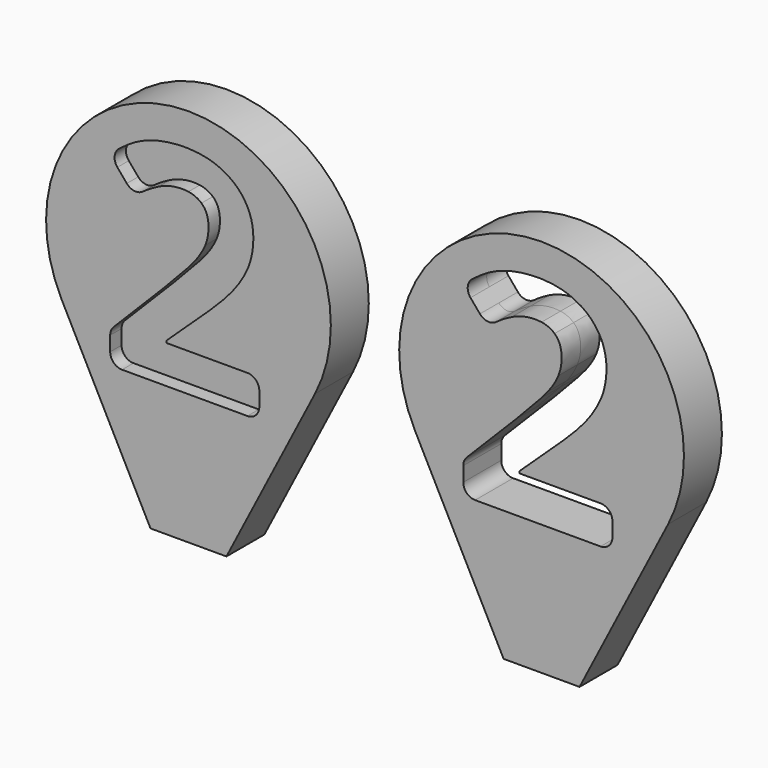
from build123d import *

# Parameters (mm, degrees)
F1_DEPTH = 3.175
F2_R     = 1.5875
F0_W     = 9.4800787622
F0_H     = 5.0789482924
F4_DEPTH = 1.27


with BuildPart() as f1:
    # F0 (on Front) → F1 (new body, symmetric)
    with BuildSketch(Plane.XZ):
        with BuildLine():
            ThreePointArc((-16.9370236714, 23.0299237874), (-9.919300584, 15.486237338), (0, 12.7))
            Line((0, 12.7), (0, 17.4584717806))
            Line((0, 17.4584717806), (-10.4733786127, 17.4584717806))
            Line((-10.4733786127, 17.4584717806), (-10.4733786127, 21.6565692621))
            Line((-10.4733786127, 21.6565692621), (-3.3078759174, 28.897037984))
            add(Edge.make_bspline(
                [(-3.3078759174, 28.897037984), (-1.1437844149, 31.1120492865), (0, 32.4033079857)],
                knots=[0, 0, 0, 0.6792383492, 0.6792383492, 0.6792383492], degree=2))
            Line((0, 32.4033079857), (0, 41.314116363))
            add(Edge.make_bspline(
                [(0, 41.314116363), (-0.3731620425, 41.3726342199), (-0.7902668622, 41.3726342199)],
                knots=[0.7360987537, 0.7360987537, 0.7360987537, 1, 1, 1], degree=2))
            add(Edge.make_bspline(
                [(-0.7902668622, 41.3726342199), (-2.4457666131, 41.3726342199), (-4.0075588309, 40.6104796177)],
                knots=[0, 0, 0, 1, 1, 1], degree=2))
            add(Edge.make_bspline(
                [(-4.0075588309, 40.6104796177), (-5.5693510488, 39.8483250154), (-7.2685809818, 38.4427120193)],
                knots=[0, 0, 0, 1, 1, 1], degree=2))
            Line((-7.2685809818, 38.4427120193), (-10.5483446392, 42.3284510573))
            add(Edge.make_bspline(
                [(-10.5483446392, 42.3284510573), (-8.4430487296, 44.1276356922), (-7.0561772401, 44.8679252034)],
                knots=[0, 0, 0, 1, 1, 1], degree=2))
            add(Edge.make_bspline(
                [(-7.0561772401, 44.8679252034), (-5.6693057507, 45.6082147147), (-4.029423922, 46.0080335225)],
                knots=[0, 0, 0, 1, 1, 1], degree=2))
            add(Edge.make_bspline(
                [(-4.029423922, 46.0080335225), (-2.3895420933, 46.4078523302), (-0.3592122101, 46.4078523302)],
                knots=[0, 0, 0, 1, 1, 1], degree=2))
            add(Edge.make_bspline(
                [(-0.3592122101, 46.4078523302), (-0.1781741178, 46.4078523302), (0, 46.40338453)],
                knots=[0, 0, 0, 0.0677084621, 0.0677084621, 0.0677084621], degree=2))
            Line((0, 46.40338453), (0, 50.8))
            ThreePointArc((0, 50.8), (-16.263762662, 41.669300584), (-16.9370236714, 23.0299237874))
        make_face()
        with BuildLine():
            add(Edge.make_bspline(
                [(1.7398365307, 40.5323900068), (1.0408594812, 41.1508927249), (0, 41.314116363)],
                knots=[0, 0, 0, 0.7360987537, 0.7360987537, 0.7360987537], degree=2))
            Line((0, 41.314116363), (0, 32.4033079857))
            add(Edge.make_bspline(
                [(0, 32.4033079857), (0.5401376078, 33.0130884441), (0.8527385509, 33.4168646624)],
                knots=[0.6792383492, 0.6792383492, 0.6792383492, 1, 1, 1], degree=2))
            add(Edge.make_bspline(
                [(0.8527385509, 33.4168646624), (1.8272968949, 34.6756691899), (2.258351547, 35.7501822358)],
                knots=[0, 0, 0, 1, 1, 1], degree=2))
            add(Edge.make_bspline(
                [(2.258351547, 35.7501822358), (2.6894061991, 36.8246952816), (2.6894061991, 37.974174354)],
                knots=[0, 0, 0, 1, 1, 1], degree=2))
            add(Edge.make_bspline(
                [(2.6894061991, 37.974174354), (2.6894061991, 39.6921457936), (1.7398365307, 40.5323900068)],
                knots=[0, 0, 0, 1, 1, 1], degree=2))
        make_face()
        with BuildLine():
            Line((0, 17.4584717806), (0, 12.7))
            ThreePointArc((0, 12.7), (9.919300584, 15.486237338), (16.9370236714, 23.0299237874))
            ThreePointArc((16.9370236714, 23.0299237874), (18.5142215734, 27.2637878417), (19.05, 31.75))
            ThreePointArc((19.05, 31.75), (13.4703841816, 45.2203841816), (0, 50.8))
            Line((0, 50.8), (0, 46.40338453))
            add(Edge.make_bspline(
                [(0, 46.40338453), (2.4533155394, 46.3418664835), (4.3636474566, 45.4332939863)],
                knots=[0.0677084621, 0.0677084621, 0.0677084621, 1, 1, 1], degree=2))
            add(Edge.make_bspline(
                [(4.3636474566, 45.4332939863), (6.4127188464, 44.4587356424), (7.5465799965, 42.7001576051)],
                knots=[0, 0, 0, 1, 1, 1], degree=2))
            add(Edge.make_bspline(
                [(7.5465799965, 42.7001576051), (8.6804411467, 40.9415795678), (8.6804411467, 38.6801044364)],
                knots=[0, 0, 0, 1, 1, 1], degree=2))
            add(Edge.make_bspline(
                [(8.6804411467, 38.6801044364), (8.6804411467, 36.7059990731), (7.987005402, 34.9786568802)],
                knots=[0, 0, 0, 1, 1, 1], degree=2))
            add(Edge.make_bspline(
                [(7.987005402, 34.9786568802), (7.2935696572, 33.2513146873), (5.8379793102, 31.4365121302)],
                knots=[0, 0, 0, 1, 1, 1], degree=2))
            add(Edge.make_bspline(
                [(5.8379793102, 31.4365121302), (4.3823889632, 29.621709573), (0.7153008358, 26.2607327203)],
                knots=[0, 0, 0, 1, 1, 1], degree=2))
            Line((0.7153008358, 26.2607327203), (0, 25.5880093152))
            Line((0, 25.5880093152), (0, 22.537420073))
            Line((0, 22.537420073), (9.4800787622, 22.537420073))
            Line((9.4800787622, 22.537420073), (9.4800787622, 17.4584717806))
            Line((9.4800787622, 17.4584717806), (0, 17.4584717806))
        make_face()
        with BuildLine():
            Line((0, 12.7), (0, 0))
            Line((0, 0), (5.08, 0))
            Line((5.08, 0), (16.9370236714, 23.0299237874))
            ThreePointArc((16.9370236714, 23.0299237874), (9.919300584, 15.486237338), (0, 12.7))
        make_face()
        with BuildLine():
            Line((-5.08, 0), (0, 0))
            Line((0, 0), (0, 12.7))
            ThreePointArc((0, 12.7), (-9.919300584, 15.486237338), (-16.9370236714, 23.0299237874))
            Line((-16.9370236714, 23.0299237874), (-5.08, 0))
        make_face()
        Polygon((-2.9580344606, 22.537420073), (0, 22.537420073), (0, 25.5880093152), (-2.9580344606, 22.8060483345), align=None)
    extrude(amount=F1_DEPTH, both=True)

    # F2
    f2_edges = [f1.edges().sort_by_distance(p)[0] for p in [
        (-10.548345, -1.5875, 42.328451),
        (-10.548345, 1.5875, 42.328451),
        (-7.268581, 1.5875, 38.442712),
        (-7.268581, -1.5875, 38.442712),
        (-10.473379, 0, 21.656569),
        (-10.473379, 0, 17.458472),
        (7.287824, 0, 43.075162),
        (9.480079, 0, 22.53742),
        (9.480079, 0, 17.458472),
    ]]
    fillet(f2_edges, radius=F2_R)


with BuildPart() as f3_1:
    # F3: copy of F1
    add(f1.part.moved(Location((47.244, 0, 0))))


with BuildPart() as f1_1:
    add(f1.part)

    # F0 (on Front) → F4 (join, symmetric)
    with BuildSketch(Plane.XZ):
        with BuildLine():
            Line((0, 41.314116363), (0, 46.40338453))
            add(Edge.make_bspline(
                [(-0.3592122101, 46.4078523302), (-0.1781741178, 46.4078523302), (0, 46.40338453)],
                knots=[0, 0, 0, 0.0677084621, 0.0677084621, 0.0677084621], degree=2))
            add(Edge.make_bspline(
                [(-4.029423922, 46.0080335225), (-2.3895420933, 46.4078523302), (-0.3592122101, 46.4078523302)],
                knots=[0, 0, 0, 1, 1, 1], degree=2))
            add(Edge.make_bspline(
                [(-7.0561772401, 44.8679252034), (-5.6693057507, 45.6082147147), (-4.029423922, 46.0080335225)],
                knots=[0, 0, 0, 1, 1, 1], degree=2))
            add(Edge.make_bspline(
                [(-10.5483446392, 42.3284510573), (-8.4430487296, 44.1276356922), (-7.0561772401, 44.8679252034)],
                knots=[0, 0, 0, 1, 1, 1], degree=2))
            Line((-10.5483446392, 42.3284510573), (-7.2685809818, 38.4427120193))
            add(Edge.make_bspline(
                [(-4.0075588309, 40.6104796177), (-5.5693510488, 39.8483250154), (-7.2685809818, 38.4427120193)],
                knots=[0, 0, 0, 1, 1, 1], degree=2))
            add(Edge.make_bspline(
                [(-0.7902668622, 41.3726342199), (-2.4457666131, 41.3726342199), (-4.0075588309, 40.6104796177)],
                knots=[0, 0, 0, 1, 1, 1], degree=2))
            add(Edge.make_bspline(
                [(0, 41.314116363), (-0.3731620425, 41.3726342199), (-0.7902668622, 41.3726342199)],
                knots=[0.7360987537, 0.7360987537, 0.7360987537, 1, 1, 1], degree=2))
        make_face()
        with BuildLine():
            Line((0, 31.75), (0, 25.5880093152))
            Line((0, 25.5880093152), (0.7153008358, 26.2607327203))
            add(Edge.make_bspline(
                [(5.8379793102, 31.4365121302), (4.3823889632, 29.621709573), (0.7153008358, 26.2607327203)],
                knots=[0, 0, 0, 1, 1, 1], degree=2))
            add(Edge.make_bspline(
                [(7.987005402, 34.9786568802), (7.2935696572, 33.2513146873), (5.8379793102, 31.4365121302)],
                knots=[0, 0, 0, 1, 1, 1], degree=2))
            add(Edge.make_bspline(
                [(8.6804411467, 38.6801044364), (8.6804411467, 36.7059990731), (7.987005402, 34.9786568802)],
                knots=[0, 0, 0, 1, 1, 1], degree=2))
            add(Edge.make_bspline(
                [(7.5465799965, 42.7001576051), (8.6804411467, 40.9415795678), (8.6804411467, 38.6801044364)],
                knots=[0, 0, 0, 1, 1, 1], degree=2))
            add(Edge.make_bspline(
                [(4.3636474566, 45.4332939863), (6.4127188464, 44.4587356424), (7.5465799965, 42.7001576051)],
                knots=[0, 0, 0, 1, 1, 1], degree=2))
            add(Edge.make_bspline(
                [(0, 46.40338453), (2.4533155394, 46.3418664835), (4.3636474566, 45.4332939863)],
                knots=[0.0677084621, 0.0677084621, 0.0677084621, 1, 1, 1], degree=2))
            Line((0, 46.40338453), (0, 41.314116363))
            add(Edge.make_bspline(
                [(1.7398365307, 40.5323900068), (1.0408594812, 41.1508927249), (0, 41.314116363)],
                knots=[0, 0, 0, 0.7360987537, 0.7360987537, 0.7360987537], degree=2))
            add(Edge.make_bspline(
                [(2.6894061991, 37.974174354), (2.6894061991, 39.6921457936), (1.7398365307, 40.5323900068)],
                knots=[0, 0, 0, 1, 1, 1], degree=2))
            add(Edge.make_bspline(
                [(2.258351547, 35.7501822358), (2.6894061991, 36.8246952816), (2.6894061991, 37.974174354)],
                knots=[0, 0, 0, 1, 1, 1], degree=2))
            add(Edge.make_bspline(
                [(0.8527385509, 33.4168646624), (1.8272968949, 34.6756691899), (2.258351547, 35.7501822358)],
                knots=[0, 0, 0, 1, 1, 1], degree=2))
            add(Edge.make_bspline(
                [(0, 32.4033079857), (0.5401376078, 33.0130884441), (0.8527385509, 33.4168646624)],
                knots=[0.6792383492, 0.6792383492, 0.6792383492, 1, 1, 1], degree=2))
            Line((0, 32.4033079857), (0, 31.75))
        make_face()
        with BuildLine():
            Line((-10.4733786127, 17.4584717806), (0, 17.4584717806))
            Line((0, 17.4584717806), (0, 22.537420073))
            Line((0, 22.537420073), (-2.9580344606, 22.537420073))
            Line((-2.9580344606, 22.537420073), (-2.9580344606, 22.8060483345))
            Line((-2.9580344606, 22.8060483345), (0, 25.5880093152))
            Line((0, 25.5880093152), (0, 31.75))
            Line((0, 31.75), (0, 32.4033079857))
            add(Edge.make_bspline(
                [(-3.3078759174, 28.897037984), (-1.1437844149, 31.1120492865), (0, 32.4033079857)],
                knots=[0, 0, 0, 0.6792383492, 0.6792383492, 0.6792383492], degree=2))
            Line((-3.3078759174, 28.897037984), (-10.4733786127, 21.6565692621))
            Line((-10.4733786127, 21.6565692621), (-10.4733786127, 17.4584717806))
        make_face()
        with Locations((4.7400393811, 19.9979459268)):
            Rectangle(F0_W, F0_H)
    extrude(amount=F4_DEPTH, both=True)


solid = Compound([f3_1.part, f1_1.part])
